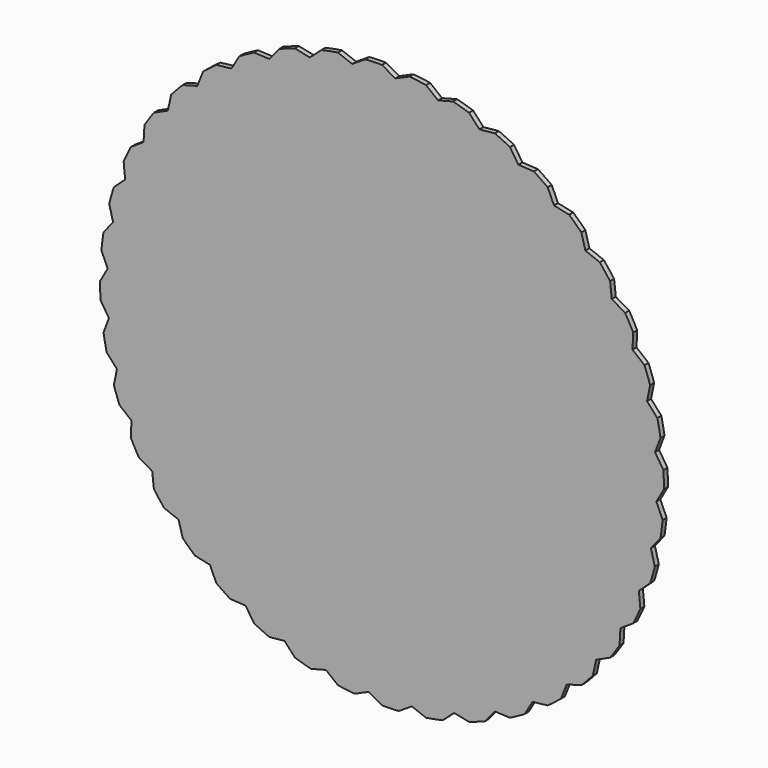
from build123d import *

# Parameters (mm, degrees)
F0_R            = 17.3228
F2_DEPTH        = 0.18542
F1_R            = 20.8153
F4_DEPTH        = 0.37184
F4_COPIES_COUNT = 40


# Not quite as in the source:
# - a feature of the source that left no trace in its solid (it failed there, or was rolled back) is left out
# - a pattern or mirror of a feature is missing from the dataset's text; its kind, count and spacing are read off the source's solid


with BuildPart() as f2:
    # F0 (on Front) → F2 (new body, symmetric)
    with BuildSketch(Plane.XZ):
        Circle(F0_R)
    extrude(amount=F2_DEPTH, both=True)


with BuildPart() as f2b:
    # F1 (on Front) → F2, piece 2 (new body, symmetric)
    with BuildSketch(Plane.XZ):
        Circle(F1_R)
    extrude(amount=F2_DEPTH, both=True)

    # F3 (on face) → F4 (cut, through all)
    with BuildSketch(Plane.XZ.offset(0.18542)):
        with BuildLine():
            ThreePointArc((2.0285952307, 20.7162138307), (1.0155068536, 20.7905137002), (0, 20.8153))
            Line((0, 20.8153), (0.9818294189, 20.2571600918))
            Line((0.9818294189, 20.2571600918), (2.0285952307, 20.7162138307))
        make_face()
    f4 = extrude(amount=-F4_DEPTH, mode=Mode.SUBTRACT)

    # F4_copies: F4 ×40 about axis
    f4_copies_axis = Axis((0, 0, 0), (0, 1, 0))
    for i in range(1, F4_COPIES_COUNT):
        add(f4.rotate(f4_copies_axis, i * 360 / F4_COPIES_COUNT), mode=Mode.SUBTRACT)


solid = Compound([f2.part, f2b.part])
